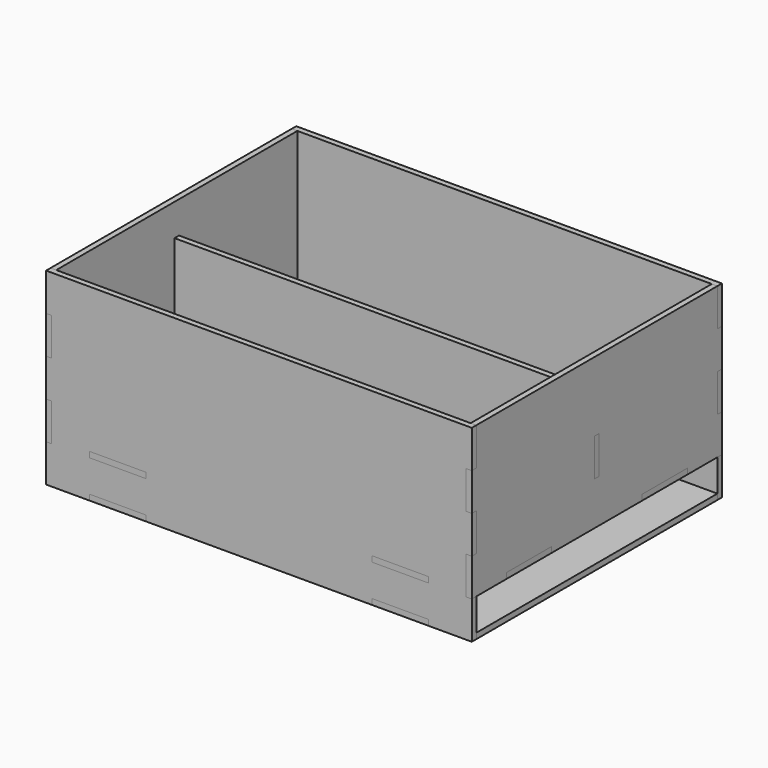
from build123d import *

# Parameters (mm, degrees)
F1_DEPTH  = 1.5
F3_DEPTH  = 3
F4_W      = 30
F4_H      = 3
F5_DEPTH  = 3
F10_DEPTH = 3
F11_W     = 60
F11_H     = 3
F11_W_2   = 20
F12_DEPTH = 3
F14_DEPTH = 1.5
F16_DEPTH = 1.5


# Not quite as in the source:
# - ends of sketch curves that miss each other by under 0.0002 mm in the source are joined


with BuildPart() as f1:
    # F0 (on Top) → F1 (new body, symmetric)
    with BuildSketch(Plane.XY):
        Polygon((-110, -60), (-110, -80), (-90, -80), (-90, -83), (-60, -83), (-60, -80), (60, -80), (60, -83), (90, -83), (90, -80), (110, -80), (110, -60), (113, -60), (113, -30), (110, -30), (110, 30), (113, 30), (113, 60), (110, 60), (110, 80), (90, 80), (90, 83), (60, 83), (60, 80), (-60, 80), (-60, 83), (-90, 83), (-90, 80), (-110, 80), (-110, 60), (-113, 60), (-113, 30), (-110, 30), (-110, -30), (-113, -30), (-113, -60), align=None)
    extrude(amount=F1_DEPTH, both=True)


with BuildPart() as f3:
    # F2 (on face) → F3 (new body)
    with BuildSketch(Plane(origin=(-110, 0, 0), x_dir=(0, -1, 0), z_dir=(-1, 0, 0))):
        Polygon((-60, 1.5), (-30, 1.5), (-30, -1.5), (30, -1.5), (30, 1.5), (60, 1.5), (60, -1.5), (80, -1.5), (80, 18.5), (83, 18.5), (83, 38.5), (80, 38.5), (80, 58.5), (82.999996841, 58.5), (82.999996841, 78.5), (79.999996841, 78.5), (79.999996841, 98.5), (-79.999996841, 98.5), (-79.999996841, 78.5), (-82.999996841, 78.5), (-82.999996841, 58.5), (-79.999996841, 58.5), (-80, 38.5), (-83, 38.5), (-83, 18.5), (-80, 18.5), (-80, -1.5), (-60, -1.5), align=None)
    extrude(amount=F3_DEPTH)


with BuildPart() as f5:
    # F4 (on face) → F5 (new body)
    with BuildSketch(Plane(origin=(0, 80, 0), x_dir=(-1, 0, 0), z_dir=(0, 1, 0))):
        Polygon((-60, -1.5), (60, -1.5), (60, 1.5), (90, 1.5), (90, -1.5), (113, -1.5), (113, 18.5), (110, 18.5), (110, 38.5), (113, 38.5), (113, 58.5), (109.999998033, 58.5), (109.999998033, 78.5), (112.999998033, 78.5), (112.999998033, 98.5), (-112.999998033, 98.5), (-112.999998033, 78.5), (-109.999998033, 78.5), (-109.999998033, 58.5), (-113, 58.5), (-113, 38.5), (-110, 38.5), (-110, 18.5), (-113, 18.5), (-113, -1.5), (-90, -1.5), (-90, 1.5), (-60, 1.5), align=None)
        with Locations((-75.0000035763, 20)):
            Rectangle(F4_W, F4_H, mode=Mode.SUBTRACT)
        with Locations((75.0000035763, 20)):
            Rectangle(F4_W, F4_H, mode=Mode.SUBTRACT)
    extrude(amount=F5_DEPTH)


with BuildPart() as f6_1:
    # F6: instance of F5
    add(f5.part.mirror(Plane.XZ))


with BuildPart() as f8_1:
    # F8: instance of F1
    add(f1.part.mirror(Plane.XY.offset(10)))


with BuildPart() as f10:
    # F9 (on face) → F10 (new body)
    with BuildSketch(Plane.YZ.offset(110)):
        Polygon((80, 98.5), (-80, 98.5), (-80, 78.5), (-83, 78.5), (-83, 58.5), (-80, 58.5), (-80, 38.5), (-83, 38.5), (-83, 18.5), (-60, 18.5), (-60, 21.5), (-30, 21.5), (-30, 18.5), (30, 18.5), (30, 21.5), (60, 21.5), (60, 18.5), (83, 18.5), (83, 38.5), (80, 38.5), (80, 58.5), (83, 58.5), (83, 78.5), (80, 78.5), align=None)
    extrude(amount=F10_DEPTH)


with BuildPart() as f1_1:
    add(f1.part)

    # F11 (on face) → F12 (join)
    with BuildSketch(Plane.YZ.offset(110)):
        Rectangle(F11_W, F11_H)
        with Locations((-70, 0)):
            Rectangle(F11_W_2, F11_H)
        with Locations((70, 0)):
            Rectangle(F11_W_2, F11_H)
    extrude(amount=F12_DEPTH)


with BuildPart() as f14_tool:
    # F13 (on Front) → F14 (new body, symmetric)
    with BuildSketch(Plane.XZ):
        Polygon((110, 61.5), (110, 81.5), (-110, 81.5), (-110, 61.5), (-113, 61.5), (-113, 41.5), (-110, 41.5), (-110, 21.5), (-90, 21.5), (-90, 18.5), (-70, 18.5), (-70, 21.5), (70, 21.5), (70, 18.5), (90, 18.5), (90, 21.5), (110, 21.5), (110, 41.5), (113, 41.5), (113, 61.5), align=None)
    extrude(amount=F14_DEPTH, both=True)


with BuildPart() as f3_1:
    add(f3.part)

    # F14: cut by f14_tool
    add(f14_tool.part, mode=Mode.SUBTRACT)


with BuildPart() as f8_1_1:
    add(f8_1.part)

    # F14: cut by f14_tool
    add(f14_tool.part, mode=Mode.SUBTRACT)


with BuildPart() as f10_1:
    add(f10.part)

    # F14: cut by f14_tool
    add(f14_tool.part, mode=Mode.SUBTRACT)


with BuildPart() as f16:
    # F15 (on Front) → F16 (new body, symmetric)
    with BuildSketch(Plane.XZ):
        Polygon((110, 81.5), (-110, 81.5), (-110, 61.5), (-113, 61.5), (-113, 41.5), (-110, 41.5), (-110, 21.5), (-90, 21.5), (-90, 18.5), (-70, 18.5), (-70, 21.5), (70, 21.5), (70, 18.5), (90, 18.5), (90, 21.5), (110, 21.5), (110, 41.5), (113, 41.5), (113, 61.5), (110, 61.5), align=None)
    extrude(amount=F16_DEPTH, both=True)


solid = Compound([f5.part, f6_1.part, f1_1.part, f3_1.part, f8_1_1.part, f10_1.part, f16.part])
